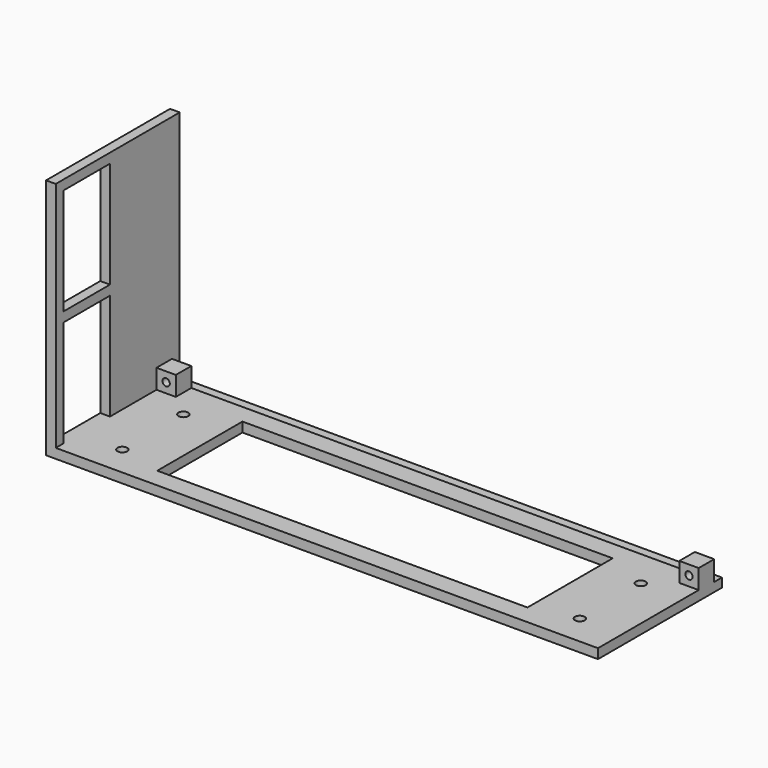
from build123d import *

# Parameters (mm, degrees)
F0_W      = 184.15
F0_H      = 50.8
F1_DEPTH  = 3.175
F3_D      = 3.2
F4_W      = 184.15
F4_H      = 3.175
F5_DEPTH  = 76.2
F7_D      = 3.3
F8_W      = 3.175
F8_H      = 47.625
F9_DEPTH  = 76.2
F10_W     = 19.05
F10_H     = 34.925
F11_DEPTH = 3.175
F12_W     = 3.175
F12_H     = 47.625
F13_DEPTH = 76.2
F14_W     = 13.2291666667
F14_H     = 31.75
F14_W_2   = 11.6416666667
F15_DEPTH = 3.175
F16_W     = 6.35
F16_H     = 6.35
F17_DEPTH = 6.35
F19_D     = 2.4
F19_DEPTH = 12.7
F19_TIP   = 0.7210327428
F20_W     = 121.4
F20_H     = 34.925
F21_DEPTH = 25.4
F22_W     = 60.2
F22_H     = 32.26
F23_DEPTH = 25.4
F24_W     = 177.8
F24_H     = 76.2
F25_DEPTH = 50.801
F26_W     = 6.35
F26_H     = 6.35
F27_DEPTH = 9.525
F28_D     = 2.4
F28_DEPTH = 12.7
F28_TIP   = 0.7210327428
F29_W     = 165.1
F29_H     = 6.35
F29_R     = 1.2
F30_DEPTH = 3.175


with BuildPart() as f1:
    # F0 (on Top) → F1 (new body)
    with BuildSketch(Plane.XY):
        with Locations((-3.8965528874, 0)):
            Rectangle(F0_W, F0_H)
    extrude(amount=F1_DEPTH)

    # F3 (through all)
    with Locations(Plane.XY.offset(3.175)):
        with Locations((-78.8965528874, 9.525), (-78.8965528874, -15.475), (71.1034471126, -15.475), (71.1034471126, 9.525)):
            Hole(F3_D / 2)

    # F4 (on face) → F5 (join)
    with BuildSketch(Plane.XY.offset(3.175)):
        with Locations((-3.8965528874, 23.8125)):
            Rectangle(F4_W, F4_H)
    extrude(amount=F5_DEPTH)

    # F7 (through all)
    with Locations(Plane.XZ.offset(-22.225)):
        with Locations((-70.5715528874, 66.675), (11.9784471126, 66.675), (10.7084471126, 18.415), (-64.2215528874, 18.415)):
            Hole(F7_D / 2)

    # F8 (on face) → F9 (join)
    with BuildSketch(Plane.XY.offset(3.175)):
        with Locations((-94.3840528874, -1.5875)):
            Rectangle(F8_W, F8_H)
    extrude(amount=F9_DEPTH)

    # F10 (on face) → F11 (cut, through all)
    with BuildSketch(Plane(origin=(-95.9715528874, 0, 0), x_dir=(0, -1, 0), z_dir=(-1, 0, 0))):
        with Locations((12.7, 58.7375)):
            Rectangle(F10_W, F10_H)
        with Locations((12.7, 20.6375)):
            Rectangle(F10_W, F10_H)
    extrude(amount=-F11_DEPTH, mode=Mode.SUBTRACT)

    # F12 (on face) → F13 (join)
    with BuildSketch(Plane.XY.offset(3.175)):
        with Locations((86.5909471126, -1.5875)):
            Rectangle(F12_W, F12_H)
    extrude(amount=F13_DEPTH)

    # F14 (on face) → F15 (cut, through all)
    with BuildSketch(Plane.YZ.offset(88.1784471126)):
        with Locations((-15.6104166667, 19.05)):
            Rectangle(F14_W, F14_H)
        with Locations((0, 19.05)):
            Rectangle(F14_W_2, F14_H)
        with Locations((15.6104166667, 19.05)):
            Rectangle(F14_W, F14_H)
    extrude(amount=-F15_DEPTH, mode=Mode.SUBTRACT)

    # F16 (on face) → F17 (join)
    with BuildSketch(Plane.XZ.offset(-22.225)):
        with Locations((-89.6215528874, 76.2)):
            Rectangle(F16_W, F16_H)
        with Locations((81.8284471126, 76.2)):
            Rectangle(F16_W, F16_H)
    extrude(amount=F17_DEPTH)

    # F19
    with Locations(Plane.XY.offset(79.375)):
        with Locations((-89.6215528874, 19.05), (81.8284471126, 19.05)):
            Hole(F19_D / 2, depth=F19_DEPTH)
            with Locations((0, 0, -(F19_DEPTH + F19_TIP / 2))):  # 118° drill point
                Cone(0, F19_D / 2, F19_TIP, mode=Mode.SUBTRACT)

    # F20 (on face) → F21 (cut)
    with BuildSketch(Plane.XY.offset(3.175)):
        with Locations((-3.8965528874, -1.5875)):
            Rectangle(F20_W, F20_H)
    extrude(amount=-F21_DEPTH, mode=Mode.SUBTRACT)

    # F22 (on face) → F23 (cut)
    with BuildSketch(Plane.XZ.offset(-22.225)):
        with Locations((-26.1215528874, 42.545)):
            Rectangle(F22_W, F22_H)
    extrude(amount=-F23_DEPTH, mode=Mode.SUBTRACT)

    # F24 (on face) → F25 (cut, through all)
    with BuildSketch(Plane.XZ.offset(25.4)):
        with Locations((-3.8965528874, 41.275)):
            Rectangle(F24_W, F24_H)
        Polygon((88.1784471126, 79.375), (85.0034471126, 79.375), (85.0034471126, 3.175), (85.0034471126, 0), (88.1784471126, 0), align=None)
    extrude(amount=-F25_DEPTH, mode=Mode.SUBTRACT)

    # F26 (on face) → F27 (join)
    with BuildSketch(Plane(origin=(0, 25.4, 0), x_dir=(-1, 0, 0), z_dir=(0, 1, 0))):
        with Locations((-81.8284471126, 6.35)):
            Rectangle(F26_W, F26_H)
        Polygon((-78.6534471126, 3.175), (-85.0034471126, 3.175), (-85.0034471126, 0), (95.9715528874, 0), (95.9715528874, 79.375), (92.7965528874, 79.375), (92.7965528874, 9.525), (92.7965528874, 3.175), (86.4465528874, 3.175), align=None)
        with Locations((89.6215528874, 6.35)):
            Rectangle(F26_W, F26_H)
    extrude(amount=-F27_DEPTH)

    # F28
    with Locations(Plane(origin=(0, 25.4, 0), x_dir=(-1, 0, 0), z_dir=(0, 1, 0))):
        with Locations((89.6215528874, 6.35), (-81.8284471126, 6.35)):
            Hole(F28_D / 2, depth=F28_DEPTH)
            with Locations((0, 0, -(F28_DEPTH + F28_TIP / 2))):  # 118° drill point
                Cone(0, F28_D / 2, F28_TIP, mode=Mode.SUBTRACT)

    # F29 (on face) → F30 (cut)
    with BuildSketch(Plane(origin=(0, 25.4, 0), x_dir=(-1, 0, 0), z_dir=(0, 1, 0))):
        with Locations((3.8965528874, 6.35)):
            Rectangle(F29_W, F29_H)
        Polygon((-78.6534471126, 9.525), (-85.0034471126, 9.525), (-85.0034471126, 2.9308686499), (92.7965528874, 2.9308686499), (92.7965528874, 9.525), (86.4465528874, 9.525), (86.4465528874, 3.175), (-78.6534471126, 3.175), align=None)
        with Locations((-81.8284471126, 6.35)):
            Circle(F29_R, mode=Mode.SUBTRACT)
        with Locations((89.6215528874, 6.35)):
            Circle(F29_R, mode=Mode.SUBTRACT)
    extrude(amount=-F30_DEPTH, mode=Mode.SUBTRACT)


solid = f1.part
